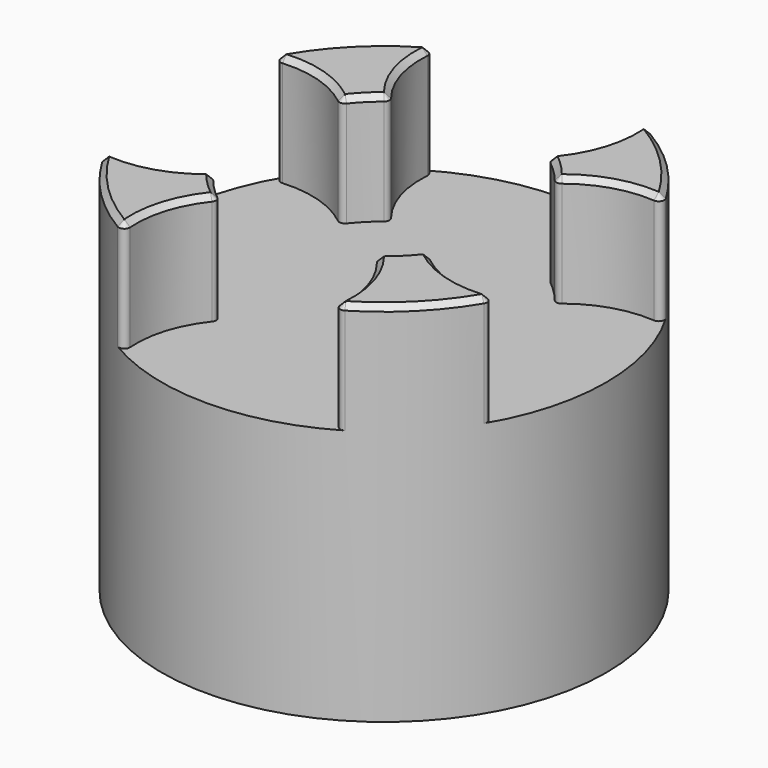
from build123d import *

# Parameters (mm, degrees)
F0_R     = 40
F1_DEPTH = 66
F2_R     = 24
F3_DEPTH = 20
F4_R     = 19
F5_DEPTH = 20
F6_R     = 1
F7_SIZE  = 0.999


# Not quite as in the source:
# - a fillet or chamfer is up to 0.001 mm smaller than in the source, because OpenCascade refuses the exact size


with BuildPart() as f1:
    # F0 (on Top) → F1 (new body)
    with BuildSketch(Plane.XY):
        Circle(F0_R)
    extrude(amount=F1_DEPTH)

    # F2 (on face) → F3 (cut)
    with BuildSketch(Plane.XY.offset(66)):
        Circle(F2_R)
    extrude(amount=-F3_DEPTH, mode=Mode.SUBTRACT)

    # F4 (on face) → F5 (cut)
    with BuildSketch(Plane.XY.offset(66)):
        with Locations((32, 0)):
            Circle(F4_R)
        with Locations((0, 32)):
            Circle(F4_R)
        with Locations((-32, 0)):
            Circle(F4_R)
        with Locations((0, -32)):
            Circle(F4_R)
    extrude(amount=-F5_DEPTH, mode=Mode.SUBTRACT)

    # F6
    f6_edges = [f1.edges().sort_by_distance(p)[0] for p in [
        (-18.700658, 35.359375, 56),
        (18.700658, 35.359375, 56),
        (35.359375, -18.700658, 56),
        (35.359375, 18.700658, 56),
        (19.359375, 14.185013, 56),
        (19.359375, -14.185013, 56),
        (14.185013, 19.359375, 56),
        (-14.185013, 19.359375, 56),
        (18.700658, -35.359375, 56),
        (-18.700658, -35.359375, 56),
        (-14.185013, -19.359375, 56),
        (14.185013, -19.359375, 56),
        (-35.359375, -18.700658, 56),
        (-35.359375, 18.700658, 56),
        (-19.359375, 14.185013, 56),
        (-19.359375, -14.185013, 56),
    ]]
    fillet(f6_edges, radius=F6_R)

    # F7 (size 1 in the source; OpenCascade refuses exactly that, so slightly less here)
    f7_edges = [f1.edges().sort_by_distance(p)[0] for p in [
        (26.400754, 18.156223, 66),
        (34.365552, 19.415588, 66),
        (19.405084, 14.631121, 66),
        (28.284271, 28.284271, 66),
        (16.970563, 16.970563, 66),
        (19.415588, 34.365552, 66),
        (14.631121, 19.405084, 66),
        (18.156223, 26.400754, 66),
        (28.284271, -28.284271, 66),
        (19.415588, -34.365552, 66),
        (34.365552, -19.415588, 66),
        (18.156223, -26.400754, 66),
        (26.400754, -18.156223, 66),
        (14.631121, -19.405084, 66),
        (19.405084, -14.631121, 66),
        (16.970563, -16.970563, 66),
        (-18.156223, 26.400754, 66),
        (-19.415588, 34.365552, 66),
        (-14.631121, 19.405084, 66),
        (-28.284271, 28.284271, 66),
        (-16.970563, 16.970563, 66),
        (-34.365552, 19.415588, 66),
        (-19.405084, 14.631121, 66),
        (-26.400754, 18.156223, 66),
        (-28.284271, -28.284271, 66),
        (-34.365552, -19.415588, 66),
        (-19.415588, -34.365552, 66),
        (-26.400754, -18.156223, 66),
        (-18.156223, -26.400754, 66),
        (-19.405084, -14.631121, 66),
        (-14.631121, -19.405084, 66),
        (-16.970563, -16.970563, 66),
    ]]
    chamfer(f7_edges, length=F7_SIZE)


solid = f1.part
